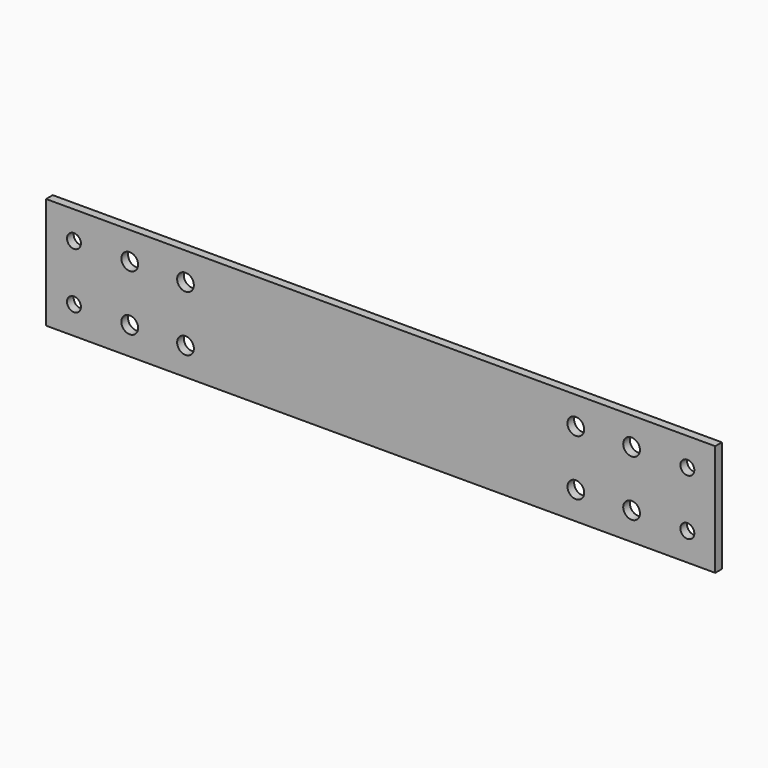
from build123d import *

# Parameters (mm, degrees)
F0_W     = 240
F0_H     = 40
F1_DEPTH = 3
F2_R     = 2.5
F3_DEPTH = 3.001
F5_R     = 3
F5_R_2   = 2.5
F6_DEPTH = 25


# Not quite as in the source:
# - a pattern or mirror of a feature is missing from the dataset's text; its kind, count and spacing are read off the source's solid


with BuildPart() as f1:
    # F0 (on Front) → F1 (new body)
    with BuildSketch(Plane.XZ):
        Rectangle(F0_W, F0_H)
    extrude(amount=F1_DEPTH)

    # F2 (on face) → F3 (cut, through all)
    with BuildSketch(Plane.XZ.offset(3)):
        with Locations((-110, 10)):
            Circle(F2_R)
        with Locations((-110, -10)):
            Circle(F2_R)
    f3 = extrude(amount=-F3_DEPTH, mode=Mode.SUBTRACT)

    # F3_copies: F3 across plane
    add(f3.mirror(Plane(origin=(0, 0, 0), x_dir=(0, 0, 1), z_dir=(1, 0, 0))), mode=Mode.SUBTRACT)

    # F5 (on face) → F6 (cut)
    with BuildSketch(Plane.XZ.offset(3)):
        with Locations((-90, 10)):
            Circle(F5_R)
        with Locations((-70, 10)):
            Circle(F5_R)
        with Locations((-70, -10)):
            Circle(F5_R)
        with Locations((-90, -10)):
            Circle(F5_R)
        with Locations((-110, -10)):
            Circle(F5_R_2)
    f6 = extrude(amount=-F6_DEPTH, mode=Mode.SUBTRACT)

    # F6_copies: F6 across plane
    add(f6.mirror(Plane(origin=(0, 0, 0), x_dir=(0, 0, 1), z_dir=(1, 0, 0))), mode=Mode.SUBTRACT)


solid = f1.part
